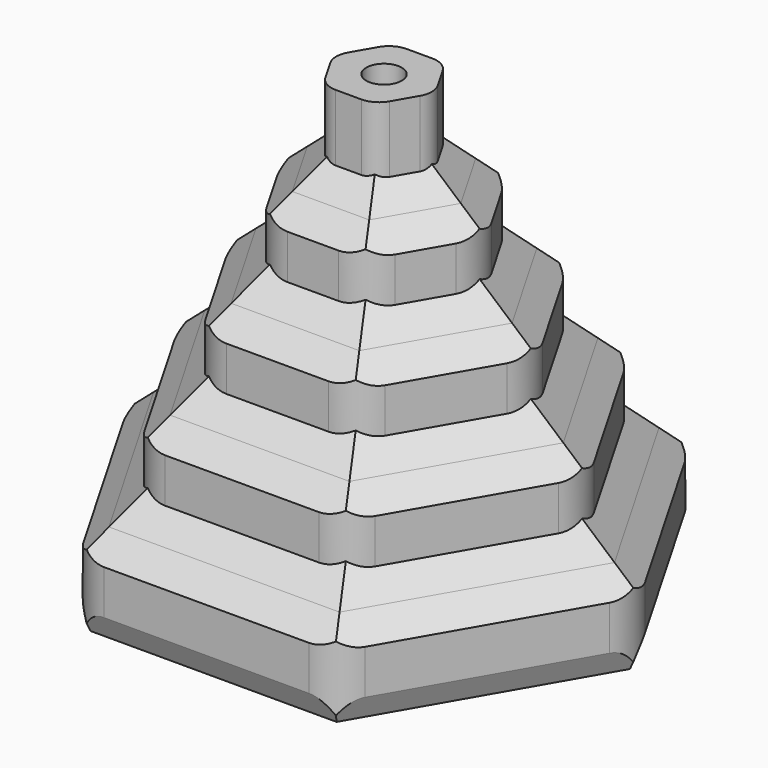
from build123d import *

# Parameters (mm, degrees)
F1_DEPTH      = 10
F3_DEPTH      = 10
F5_DEPTH      = 10
F7_DEPTH      = 10
F9_DEPTH      = 10
F10_SIZE2     = 2.5
F10_SIZE      = 1
F11_R         = 2.5
F11_TEXT_SIZE = 11.1111111111
F12_DEPTH     = 1
F13_R         = 2
F14_DEPTH     = 50.001
F15_SIZE      = 2.49999
F16_R         = 5
F17_R         = 2.5


# Not quite as in the source:
# - a fillet or chamfer is up to 0.001 mm smaller than in the source, because OpenCascade refuses the exact size
# - Text() gives the source's letters only with a copy of the font that has no kerning and outlines rounded to 1/6400 em; it was checked with that copy


with BuildPart() as f1:
    # F0 (on Top) → F1 (new body)
    with BuildSketch(Plane.XY):
        Polygon((14.4337567297, 25), (-14.4337567297, 25), (-28.8675134595, 0), (-14.4337567297, -25), (14.4337567297, -25), (28.8675134595, 0), align=None)
    extrude(amount=F1_DEPTH)

    # F2 (on face) → F3 (join)
    with BuildSketch(Plane.XY.offset(10)):
        Polygon((11.5470053838, 20), (-11.5470053838, 20), (-23.0940107676, 0), (-11.5470053838, -20), (11.5470053838, -20), (23.0940107676, 0), align=None)
    extrude(amount=F3_DEPTH)

    # F4 (on face) → F5 (join)
    with BuildSketch(Plane.XY.offset(20)):
        Polygon((8.6602540378, 15), (-8.6602540378, 15), (-17.3205080757, 0), (-8.6602540378, -15), (8.6602540378, -15), (17.3205080757, 0), align=None)
    extrude(amount=F5_DEPTH)

    # F6 (on face) → F7 (join)
    with BuildSketch(Plane.XY.offset(30)):
        Polygon((5.7735026919, 10), (-5.7735026919, 10), (-11.5470053838, 0), (-5.7735026919, -10), (5.7735026919, -10), (11.5470053838, 0), align=None)
    extrude(amount=F7_DEPTH)

    # F8 (on face) → F9 (join)
    with BuildSketch(Plane.XY.offset(40)):
        Polygon((2.8867513459, 5), (-2.8867513459, 5), (-5.7735026919, 0), (-2.8867513459, -5), (2.8867513459, -5), (5.7735026919, 0), align=None)
    extrude(amount=F9_DEPTH)

    # F10
    f10_edges = [f1.edges().sort_by_distance(p)[0] for p in [
        (21.650635, 12.5, 0),
        (0, 25, 0),
        (-21.650635, 12.5, 0),
        (-21.650635, -12.5, 0),
        (0, -25, 0),
        (21.650635, -12.5, 0),
    ]]
    f10_side = f1.faces().sort_by_distance((0, 0, 0))[0]
    chamfer(f10_edges, length=F10_SIZE, length2=F10_SIZE2, reference=f10_side)

    # F11 (on face) → F12 (cut)
    with BuildSketch(Plane(origin=(0, 0, 0), x_dir=(1, 0, 0), z_dir=(0, 0, -1))):
        Circle(F11_R)
        with Locations((-3.3090277778, 11)):
            Text('Z', F11_TEXT_SIZE, font='Open Sans', text_align=(TextAlign.LEFT, TextAlign.BOTTOM))
        with Locations((8.4548611111, -12)):
            Text('X', F11_TEXT_SIZE, font='Open Sans', text_align=(TextAlign.LEFT, TextAlign.BOTTOM))
        with Locations((-15.4713541667, -12)):
            Text('Y', F11_TEXT_SIZE, font='Open Sans', text_align=(TextAlign.LEFT, TextAlign.BOTTOM))
    extrude(amount=-F12_DEPTH, mode=Mode.SUBTRACT)

    # F13 (on face) → F14 (cut, through all)
    with BuildSketch(Plane.XY.offset(50)):
        Circle(F13_R)
    extrude(amount=-F14_DEPTH, mode=Mode.SUBTRACT)

    # F15 (size 2.5 in the source; OpenCascade refuses exactly that, so slightly less here)
    f15_edges = [f1.edges().sort_by_distance(p)[0] for p in [
        (21.650635, 12.5, 10),
        (21.650635, -12.5, 10),
        (0, 25, 10),
        (0, -25, 10),
        (-21.650635, 12.5, 10),
        (-21.650635, -12.5, 10),
        (0, 20, 10),
        (-17.320508, 10, 10),
        (-17.320508, -10, 10),
        (0, -20, 10),
        (17.320508, -10, 10),
        (17.320508, 10, 10),
        (0, 20, 20),
        (17.320508, 10, 20),
        (-17.320508, 10, 20),
        (17.320508, -10, 20),
        (-17.320508, -10, 20),
        (0, -20, 20),
        (0, 15, 20),
        (-12.990381, 7.5, 20),
        (-12.990381, -7.5, 20),
        (0, -15, 20),
        (12.990381, -7.5, 20),
        (12.990381, 7.5, 20),
        (0, 15, 30),
        (12.990381, 7.5, 30),
        (-12.990381, 7.5, 30),
        (12.990381, -7.5, 30),
        (-12.990381, -7.5, 30),
        (0, -15, 30),
        (8.660254, 5, 30),
        (0, 10, 30),
        (-8.660254, 5, 30),
        (-8.660254, -5, 30),
        (0, -10, 30),
        (8.660254, -5, 30),
        (8.660254, 5, 40),
        (8.660254, -5, 40),
        (0, 10, 40),
        (0, -10, 40),
        (-8.660254, 5, 40),
        (-8.660254, -5, 40),
        (0, 5, 40),
        (-4.330127, 2.5, 40),
        (-4.330127, -2.5, 40),
        (0, -5, 40),
        (4.330127, -2.5, 40),
        (4.330127, 2.5, 40),
    ]]
    chamfer(f15_edges, length=F15_SIZE)

    # F16
    f16_edges = [f1.edges().sort_by_distance(p)[0] for p in [
        (14.433757, -25, 5.000005),
        (28.867513, 0, 5.000005),
        (14.433757, 25, 5.000005),
        (-14.433757, 25, 5.000005),
        (-28.867513, 0, 5.000005),
        (-14.433757, -25, 5.000005),
        (-11.547005, -20, 15),
        (11.547005, -20, 15),
        (23.094011, 0, 15),
        (11.547005, 20, 15),
        (-11.547005, 20, 15),
        (-23.094011, 0, 15),
        (8.660254, -15, 25),
        (-8.660254, -15, 25),
        (17.320508, 0, 25),
        (8.660254, 15, 25),
        (-8.660254, 15, 25),
        (-17.320508, 0, 25),
        (-11.547005, 0, 35),
        (-5.773503, 10, 35),
        (5.773503, 10, 35),
        (11.547005, 0, 35),
        (5.773503, -10, 35),
        (-5.773503, -10, 35),
    ]]
    fillet(f16_edges, radius=F16_R)

    # F17
    f17_edges = [f1.edges().sort_by_distance(p)[0] for p in [
        (2.886751, -5, 46.249995),
        (5.773503, 0, 46.249995),
        (2.886751, 5, 46.249995),
        (-2.886751, 5, 46.249995),
        (-5.773503, 0, 46.249995),
        (-2.886751, -5, 46.249995),
    ]]
    fillet(f17_edges, radius=F17_R)


solid = f1.part
